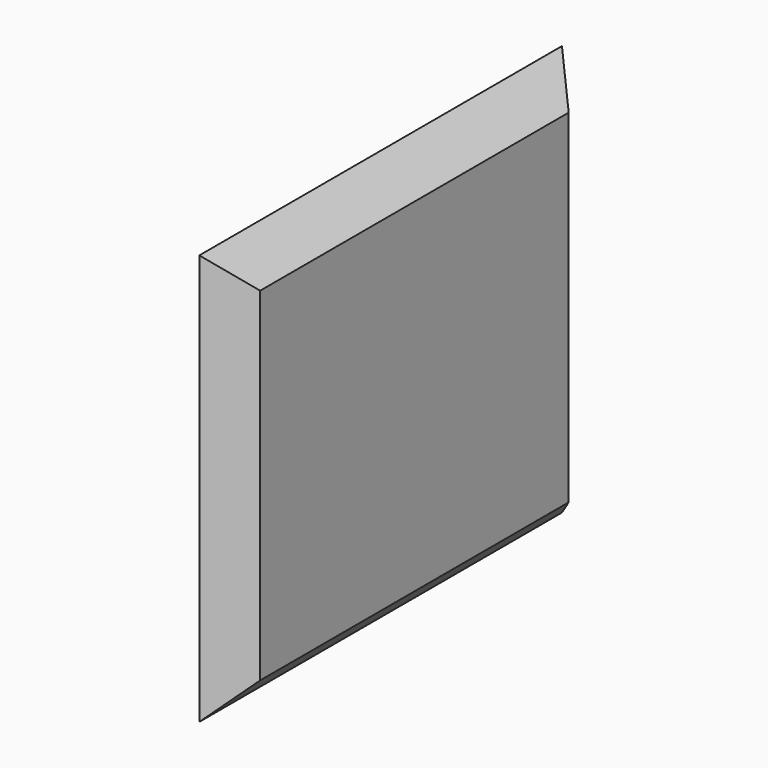
from build123d import *

# Parameters (mm, degrees)
F0_W     = 114.0731200576
F0_H     = 101.4817282557
F1_DEPTH = 10
F1_TAPER = -45
F2_W     = 32.8839123249
F2_H     = 35.4949785396
F3_DEPTH = 25


with BuildPart() as f1:
    # F0 (on Right) → F1 (new body)
    with BuildSketch(Plane.YZ):
        with Locations((23.8430835307, 1.4738403261)):
            Rectangle(F0_W, F0_H)
    extrude(amount=-F1_DEPTH, taper=F1_TAPER)

    # F2 (on face) → F3 (join)
    with BuildSketch(Plane.YZ):
        with Locations((-2.8988905251, -20.2437178232)):
            Rectangle(F2_W, F2_H)
    extrude(amount=-F3_DEPTH)


solid = f1.part
